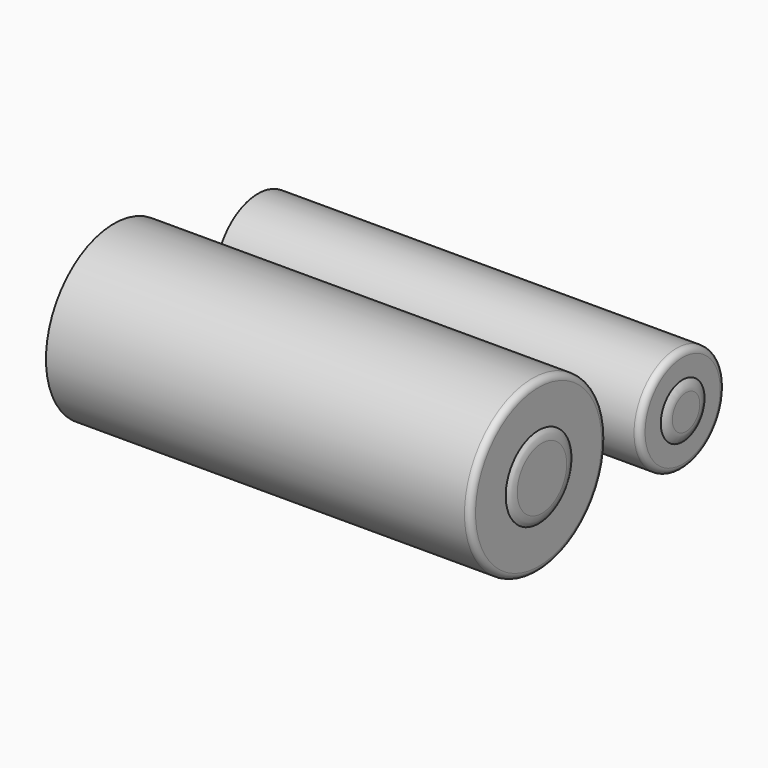
from build123d import *

# Parameters (mm, degrees)
F0_R     = 2.54
F1_DEPTH = 12.7
F0_R_2   = 1.5875
F2_R     = 0.1839630735
F2_2_R   = 0.1839630735
F3_R     = 1.2288024755
F4_DEPTH = 0.1016
F5_R     = 0.8173198651
F6_DEPTH = 0.1016


# Not quite as in the source:
# - a fillet or chamfer that OpenCascade refuses, or shapes differently, is made with other operations: its cross-section is extruded or revolved along the edge and cut away or added
# - a feature names something its author has since deleted; it is built from what else it names


with BuildPart() as f1:
    # F0 (on Right) → F1 (new body)
    with BuildSketch(Plane.YZ):
        with Locations((-44.8044711261, 24.6045570821)):
            Circle(F0_R)
    extrude(amount=F1_DEPTH)

    # F2
    f2_edges = [f1.edges().sort_by_distance(p)[0] for p in [
        (12.7, -47.344471, 24.604557),
    ]]
    fillet(f2_edges, radius=F2_R)


with BuildPart() as f1b:
    # F0 (on Right) → F1, piece 2 (new body)
    with BuildSketch(Plane.YZ):
        with Locations((-39.4185185432, 24.1574086249)):
            Circle(F0_R_2)
    extrude(amount=F1_DEPTH)

    # F2#2
    f2_2_edges = [f1b.edges().sort_by_distance(p)[0] for p in [
        (12.7, -41.006019, 24.157409),
    ]]
    fillet(f2_2_edges, radius=F2_2_R)

    # F5 (on face) → F6 (join)
    with BuildSketch(Plane.YZ.offset(12.7)):
        with Locations((-39.4185185432, 24.1574086249)):
            Circle(F5_R)
    extrude(amount=F6_DEPTH)

    # F7: fillet of radius 0.508 on 1 edges, made by hand

    # F7_s1 → F7_t2 (revolve, cut)
    with BuildSketch(Plane.XY.offset(24.1574086249)):
        with BuildLine():
            ThreePointArc((12.7, -38.6011986781), (12.7755311154, -38.745354973), (12.8016, -38.9059986781))
            Line((12.8016, -38.9059986781), (12.8016, -38.6011986781))
            Line((12.8016, -38.6011986781), (12.7, -38.6011986781))
        make_face()
    revolve(axis=Axis((12.8016, -39.4185185432, 24.1574086249), (1, 0, 0)), mode=Mode.SUBTRACT)


with BuildPart() as f4:
    # F3 (on face) → F4 (new body)
    with BuildSketch(Plane.YZ.offset(12.7)):
        with Locations((-44.8044711261, 24.6045570821)):
            Circle(F3_R)
    extrude(amount=F4_DEPTH)

    # F7#2: fillet of radius 0.508 on 1 edges, made by hand

    # F7_2_s1 → F7_2_t2 (revolve, cut)
    with BuildSketch(Plane.XY.offset(24.6045570821)):
        with BuildLine():
            ThreePointArc((12.7, -43.5756686507), (12.7755311154, -43.7198249455), (12.8016, -43.8804686507))
            Line((12.8016, -43.8804686507), (12.8016, -43.5756686507))
            Line((12.8016, -43.5756686507), (12.7, -43.5756686507))
        make_face()
    revolve(axis=Axis((12.8016, -44.8044711261, 24.6045570821), (1, 0, 0)), mode=Mode.SUBTRACT)


solid = Compound([f1.part, f1b.part, f4.part])
